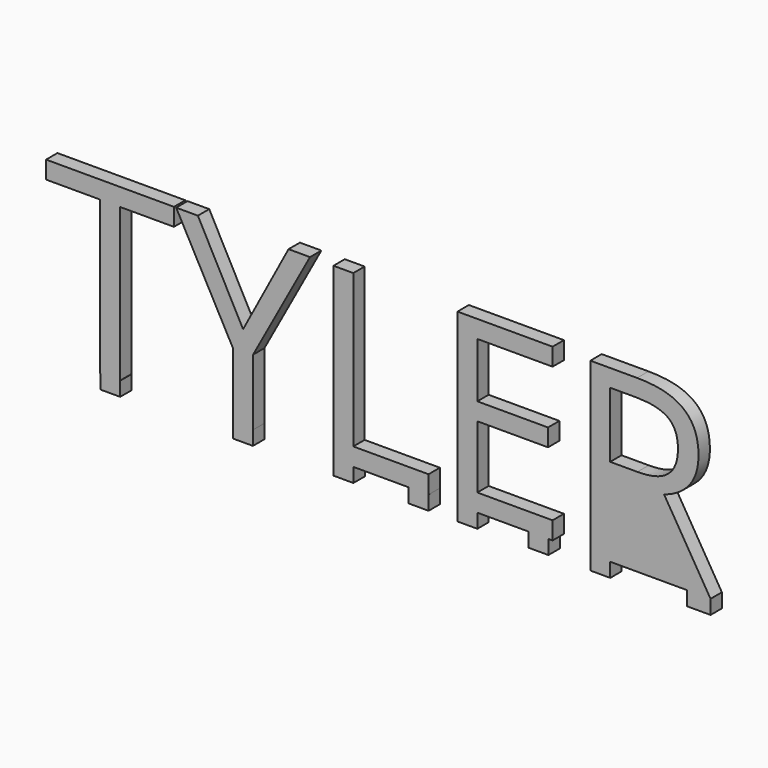
from build123d import *

# Parameters (mm, degrees)
F0_W         = 8.89
F0_H         = 6.35
F0_TEXT_SIZE = 106.7834464638
F1_DEPTH     = 6.35


# Not quite as in the source:
# - ends of sketch curves that miss each other by under 0.0002 mm in the source are joined
# - Text() gives the source's letters only with a copy of the font that has no kerning and outlines rounded to 1/6400 em; it was checked with that copy


with BuildPart() as f1:
    # F0 (on Front) → F1 (new body)
    with BuildSketch(Plane.XZ):
        Polygon((-41.8687090278, -18.3536739612), (-42.1176999807, -18.3536739612), (-42.1176999807, -24.7036739612), (-33.2276999807, -24.7036739612), (-33.2276999807, -18.3536739612), (-33.2813151181, -18.3536739612), align=None)
        Polygon((126.4576286221, -18.3536739612), (160.7932299376, -18.3536739612), (160.7935547504, -18.3536739612), (142.3400404083, 13.3476617077), (126.4226329198, 13.3476617077), (126.4226329198, -18.3536739612), (126.4237761497, -18.3536739612), align=None)
        Polygon((160.7935547504, -18.3536739612), (160.7932299376, -18.3536739612), (160.7932299376, -24.7036739612), (171.2834299376, -24.7036739612), (171.2834299376, -18.3536739612), (171.2716804346, -18.3536739612), (171.2574064732, -18.3536739612), align=None)
        Polygon((126.4576286221, -24.7036739612), (126.4576286221, -18.3536739612), (126.4237761497, -18.3536739612), (126.4226329198, -18.3536739612), (117.5676286221, -18.3536739612), (117.5676286221, -24.7036739612), align=None)
        Polygon((-92.8646251559, -18.3536739612), (-101.4520153403, -18.3536739612), (-101.4520153403, -24.7036739612), (-92.5620153403, -24.7036739612), (-92.5620153403, -18.3536739612), (-92.6669663795, -18.3536739612), align=None)
        with Locations((7.2218560685, -21.5286739612)):
            Rectangle(F0_W, F0_H)
        Polygon((42.588416487, -18.3536739612), (36.374475807, -18.3536739612), (36.374475807, -24.7036739612), (45.264475807, -24.7036739612), (45.264475807, -18.3536739612), (45.2505286939, -18.3536739612), align=None)
        Polygon((58.1813366641, -18.3536739612), (58.1673681736, -18.3536739612), (58.1673681736, -24.7036739612), (67.0573681736, -24.7036739612), (67.0573681736, -18.3536739612), align=None)
        with Locations((-126.6040804587, -18.3536739612)):
            Text('TYLER', F0_TEXT_SIZE, font='Open Sans', text_align=(TextAlign.LEFT, TextAlign.BOTTOM))
        with Locations((94.3800345135, -21.5286739612)):
            Rectangle(F0_W, F0_H)
    extrude(amount=-F1_DEPTH)


solid = f1.part
